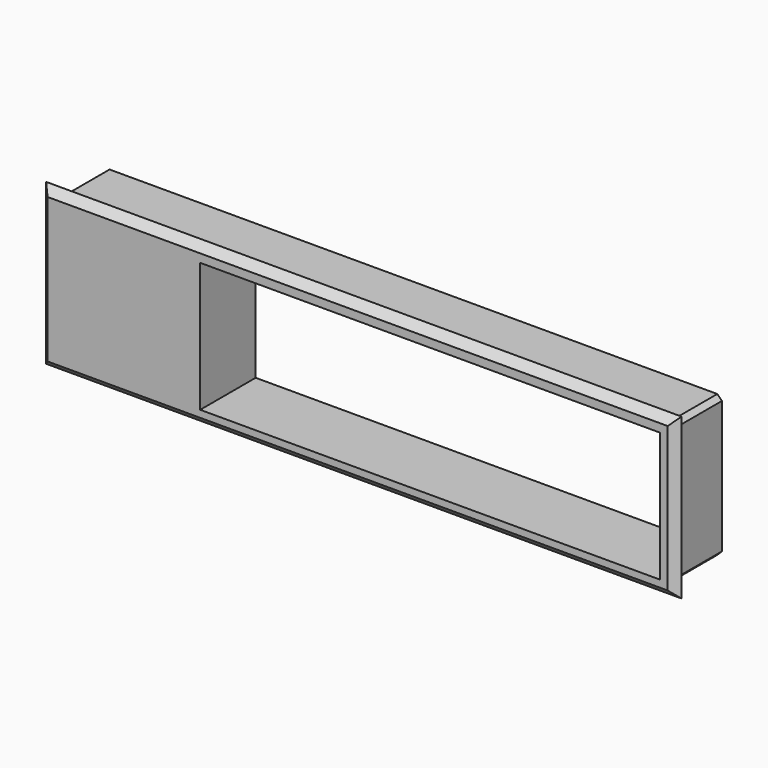
from build123d import *

# Parameters (mm, degrees)
F0_W      = 206.3
F0_H      = 52
F1_DEPTH  = 2.5
F2_SIZE   = 2.49999
F3_W      = 200.3
F3_H      = 46
F4_DEPTH  = 20
F5_W      = 196.3
F5_H      = 42
F6_DEPTH  = 25
F7_SIZE   = 1.5
F8_DEPTH  = 47
F9_W      = 43.8446728513
F9_H      = 40.8840479795
F10_DEPTH = 20.5


# Not quite as in the source:
# - a fillet or chamfer is up to 0.001 mm smaller than in the source, because OpenCascade refuses the exact size


with BuildPart() as f1:
    # F0 (on Front) → F1 (new body)
    with BuildSketch(Plane.XZ):
        with Locations((81.9657886937, 18.1555162981)):
            Rectangle(F0_W, F0_H)
    extrude(amount=F1_DEPTH)

    # F2 (size 2.5 in the source; OpenCascade refuses exactly that, so slightly less here)
    f2_edges = [f1.edges().sort_by_distance(p)[0] for p in [
        (81.965789, -2.5, 44.155516),
        (81.965789, -2.5, -7.844484),
        (185.115789, -2.5, 18.155516),
        (-21.184211, -2.5, 18.155516),
    ]]
    chamfer(f2_edges, length=F2_SIZE)

    # F3 (on face) → F4 (join)
    with BuildSketch(Plane(origin=(0, 0, 0), x_dir=(-1, 0, 0), z_dir=(0, 1, 0))):
        with Locations((-82.0777288884, 18.0567920078)):
            Rectangle(F3_W, F3_H)
    extrude(amount=F4_DEPTH)

    # F5 (on face) → F6 (cut)
    with BuildSketch(Plane(origin=(0, 20, 0), x_dir=(-1, 0, 0), z_dir=(0, 1, 0))):
        with Locations((-82.0056978608, 17.9472315861)):
            Rectangle(F5_W, F5_H)
    extrude(amount=-F6_DEPTH, mode=Mode.SUBTRACT)

    # F7
    f7_edges = [f1.edges().sort_by_distance(p)[0] for p in [
        (182.227729, 10, 41.056792),
        (182.227729, 10, -4.943208),
        (-18.072271, 10, 41.056792),
        (-18.072271, 10, -4.943208),
    ]]
    chamfer(f7_edges, length=F7_SIZE)

    # F8 (add): a face of the model
    f8_faces = [f1.faces().sort_by_distance(p)[0] for p in [
        (-16.1443021392, 8.75, 17.9472315861),
    ]]
    extrude(f8_faces, amount=F8_DEPTH)

    # F9 (on face) → F10 (cut)
    with BuildSketch(Plane(origin=(0, 20, 0), x_dir=(-1, 0, 0), z_dir=(0, 1, 0))):
        with Locations((-6.3970577903, 18.1101224152)):
            Rectangle(F9_W, F9_H)
    extrude(amount=-F10_DEPTH, mode=Mode.SUBTRACT)


solid = f1.part
